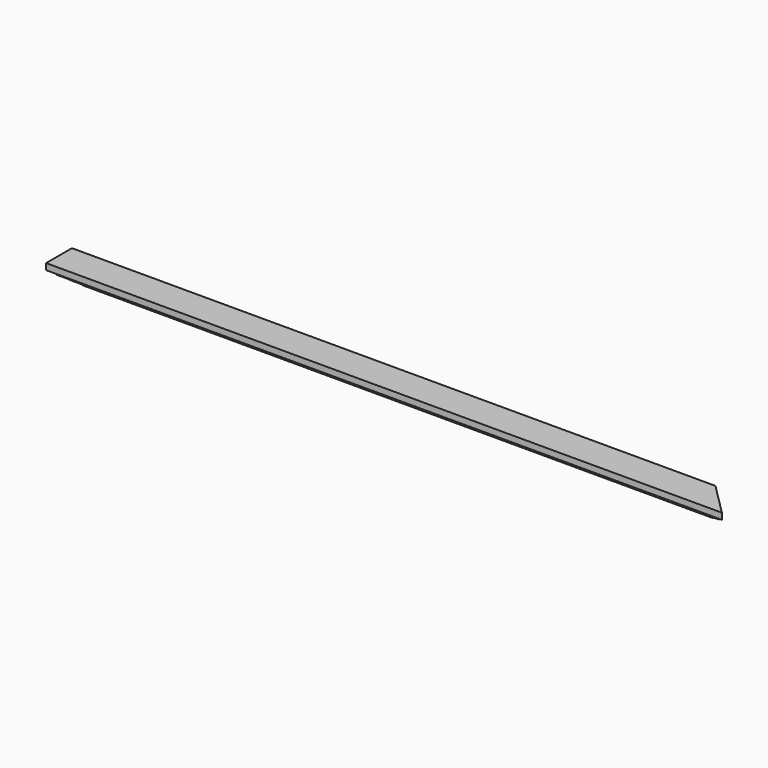
from build123d import *

# Parameters (mm, degrees)
F1_DEPTH      = 177.8
F1_DEPTH_BACK = 228.6
F3_DEPTH      = 36.7586830666


# Not quite as in the source:
# - a feature names something its author has since deleted; it is built from what else it names


with BuildPart() as f1:
    # F0 (on Right) → F1 (new body, two sides)
    with BuildSketch(Plane.YZ) as f1_sk:
        with BuildLine():
            Line((0, 0), (0, 7.62))
            Line((0, 7.62), (-41.6129238499, 36.7576829666))
            Line((-41.6129238499, 36.7576829666), (-59.6469238499, 36.7576829666))
            Line((-59.6469238499, 36.7576829666), (-59.6469238499, 33.2651829666))
            Line((-59.6469238499, 33.2651829666), (-55.5780977011, 33.2651829666))
            add(Edge.make_bspline(
                [(-45.6326596341, 29.6676454746), (-49.8473398191, 25.4529652896), (-53.5381393586, 29.571723151), (-52.9344401232, 28.3239668416), (-55.5780977011, 33.2651829666)],
                knots=[0, 0, 0, 0, 0.5235508263, 1, 1, 1, 1], degree=3))
            add(Edge.make_bspline(
                [(-45.6326596341, 29.6676454746), (-44.9426054856, 18.9718303883), (-39.7672124109, 18.9718303883), (-36.6619780561, 25.6998443657)],
                knots=[0, 0, 0, 0, 9.8090047208, 9.8090047208, 9.8090047208, 9.8090047208], degree=3))
            Line((-36.6619780561, 25.6998443657), (-34.1559106391, 15.4807388001))
            Line((-34.1559106391, 15.4807388001), (-29.0110725909, 17.0878581703))
            add(Edge.make_bspline(
                [(-10.668, 0), (-11.1556913461, 2.7848342744), (-10.6612735812, 5.9386353992), (-12.9440118592, 8.7641226677), (-27.9097380346, 10.3951310482), (-29.0110725909, 17.0878581703)],
                knots=[0, 0, 0, 0, 0.2878148332, 0.4945394705, 1, 1, 1, 1], degree=3))
            Line((-10.668, 0), (0, 0))
        make_face()
    extrude(amount=F1_DEPTH)
    extrude(f1_sk.sketch, amount=-F1_DEPTH_BACK)

    # F2 (on Top) → F3 (cut, through all)
    with BuildSketch(Plane.XY):
        Polygon((184.1130062819, 0), (88.9, 0), (184.1130062819, -95.2130062819), align=None)
    extrude(amount=F3_DEPTH, mode=Mode.SUBTRACT)


solid = f1.part
